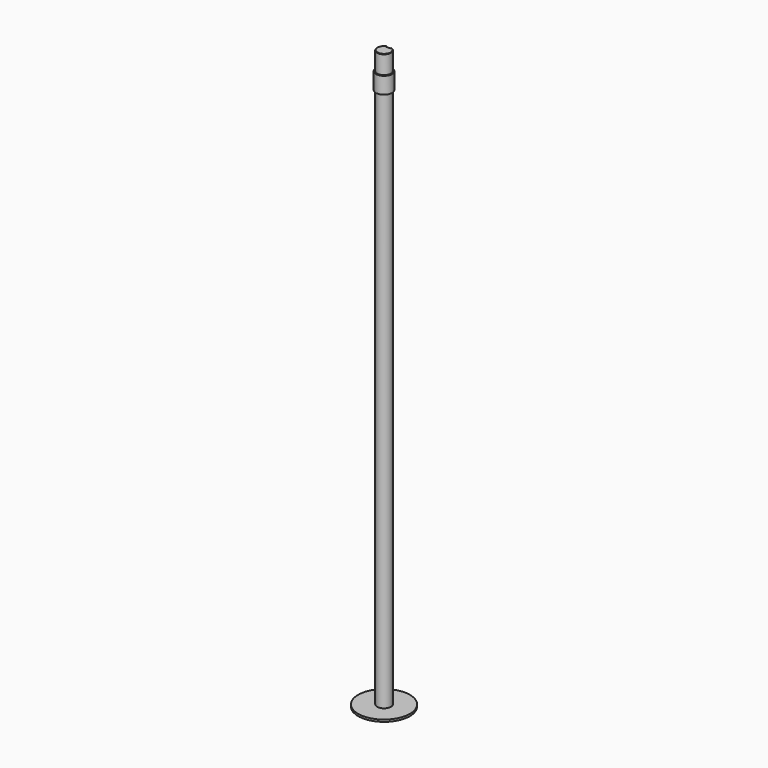
from build123d import *

# Parameters (mm, degrees)
F0_R      = 20
F1_DEPTH  = 1672
F2_R      = 75
F3_DEPTH  = 6
F5_R      = 23.5
F6_DEPTH  = 48
F7_R      = 0.5
F8_R      = 1
F9_W      = 12
F9_H      = 5
F10_DEPTH = 45
F11_R     = 4.99999
F12_SIZE2 = 1
F12_SIZE  = 1


# Not quite as in the source:
# - a fillet or chamfer is up to 0.001 mm smaller than in the source, because OpenCascade refuses the exact size


with BuildPart() as f1:
    # F0 (on Top) → F1 (new body)
    with BuildSketch(Plane.XY):
        Circle(F0_R)
    extrude(amount=F1_DEPTH)

    # F2 (on face) → F3 (join)
    with BuildSketch(Plane(origin=(0, 0, 0), x_dir=(1, 0, 0), z_dir=(0, 0, -1))):
        Circle(F2_R)
    extrude(amount=F3_DEPTH)

    # F5 (on offset) → F6 (join)
    with BuildSketch(Plane.XY.offset(1569.91401)):
        Circle(F5_R)
    extrude(amount=F6_DEPTH)

    # F7
    f7_edges = [f1.edges().sort_by_distance(p)[0] for p in [
        (-20, 0, 1617.91401),
    ]]
    fillet(f7_edges, radius=F7_R)

    # F8
    f8_edges = [f1.edges().sort_by_distance(p)[0] for p in [
        (-20, 0, 1569.91401),
    ]]
    fillet(f8_edges, radius=F8_R)

    # F9 (on face) → F10 (cut)
    with BuildSketch(Plane.XY.offset(1672)):
        with Locations((0, 17.5)):
            Rectangle(F9_W, F9_H)
    extrude(amount=-F10_DEPTH, mode=Mode.SUBTRACT)

    # F11 (radius 5 in the source; OpenCascade refuses exactly that, so slightly less here)
    f11_edges = [f1.edges().sort_by_distance(p)[0] for p in [
        (0, 15, 1627),
    ]]
    fillet(f11_edges, radius=F11_R)

    # F12
    f12_edges = [f1.edges().sort_by_distance(p)[0] for p in [
        (-11.83216, -16.124515, 1672),
    ]]
    chamfer(f12_edges, length=F12_SIZE, length2=F12_SIZE2)


solid = f1.part
